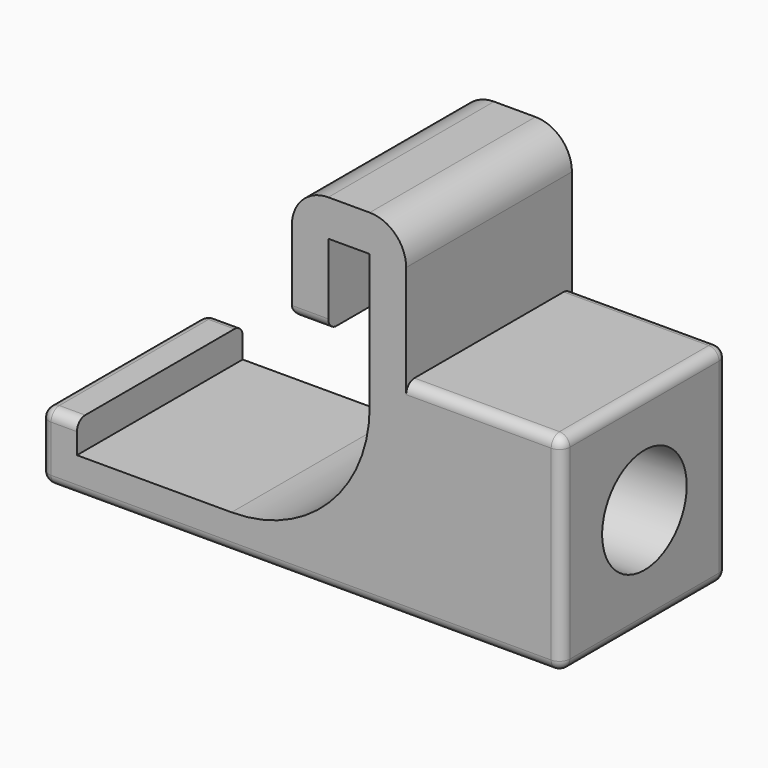
from build123d import *

# Parameters (mm, degrees)
F1_DEPTH = 20
F2_DEPTH = 20
F3_W     = 20
F3_H     = 20
F4_DEPTH = 15
F5_R     = 5.1
F6_DEPTH = 15
F7_R     = 1


# Not quite as in the source:
# - a feature names something its author has since deleted; it is built from what else it names


with BuildPart() as f1:
    # F0 (on Front) → F1 (new body)
    with BuildSketch(Plane.XZ):
        with BuildLine():
            Line((-11.0182737141, 21.9913642435), (-7.5182737801, 21.9906845019))
            Line((-7.5182737801, 21.9906845019), (-7.5182737801, 29.8039734362))
            Line((-7.5182737801, 29.8039734362), (-3.5182737801, 29.8039734362))
            Line((-3.5182737801, 29.8039734362), (-3.5182737801, 16.8525947745))
            ThreePointArc((-3.5182737801, 16.8525947745), (-7.4238059768, 7.4238059768), (-16.8525947745, 3.5182737801))
            Line((-16.8525947745, 3.5182737801), (-31.7764421987, 3.5182737801))
            Line((-31.7764421987, 3.5182737801), (-31.7764421987, 6.5182737801))
            Line((-31.7764421987, 6.5182737801), (-35.2764421987, 6.5182737801))
            Line((-35.2764421987, 6.5182737801), (-35.2764421987, 0))
            Line((-35.2764421987, 0), (-16.8525947745, 0))
            ThreePointArc((-16.8525947745, 0), (-4.9360107289, 4.9360107289), (0, 16.8525947745))
            Line((0, 16.8525947745), (0, 29.8039734362))
            ThreePointArc((0, 29.8039734362), (-1.0304785321, 32.2917686842), (-3.5182737801, 33.3222472163))
            Line((-3.5182737801, 33.3222472163), (-7.5182737801, 33.3222472163))
            ThreePointArc((-7.5182737801, 33.3222472163), (-10.0040648606, 32.2914241533), (-11.0308766315, 29.8039734362))
            Line((-11.0308766315, 29.8039734362), (-11.0182737141, 21.9913642435))
        make_face()
    extrude(amount=F1_DEPTH)

    # F0 (on Front) → F2 (join)
    with BuildSketch(Plane.XZ):
        with BuildLine():
            Line((0, 0), (0, 16.8525947745))
            ThreePointArc((0, 16.8525947745), (-4.9360107289, 4.9360107289), (-16.8525947745, 0))
            Line((-16.8525947745, 0), (0, 0))
        make_face()
    extrude(amount=F2_DEPTH)

    # F3 (on face) → F4 (join)
    with BuildSketch(Plane.YZ):
        with Locations((-10, 10)):
            Rectangle(F3_W, F3_H)
    extrude(amount=F4_DEPTH)

    # F5 (on face) → F6 (cut)
    with BuildSketch(Plane.YZ.offset(15)):
        with Locations((-10, 10)):
            Circle(F5_R)
    extrude(amount=-F6_DEPTH, mode=Mode.SUBTRACT)

    # F7
    f7_edges = [f1.edges().sort_by_distance(p)[0] for p in [
        (-10.138221, -20, 0),
        (-10.138221, 0, 0),
        (-35.276442, -10, 0),
        (-35.276442, -10, 6.518274),
        (-35.276442, 0, 3.259137),
        (-35.276442, -20, 3.259137),
        (-33.526442, -20, 6.518274),
        (-33.526442, 0, 6.518274),
        (-9.268274, 0, 21.991024),
        (-9.268274, -20, 21.991024),
        (-11.018274, -10, 21.991364),
        (7.5, 0, 20),
        (7.5, -20, 20),
        (15, 0, 10),
        (15, -10, 20),
        (15, -20, 10),
        (15, -10, 0),
    ]]
    fillet(f7_edges, radius=F7_R)


solid = f1.part
